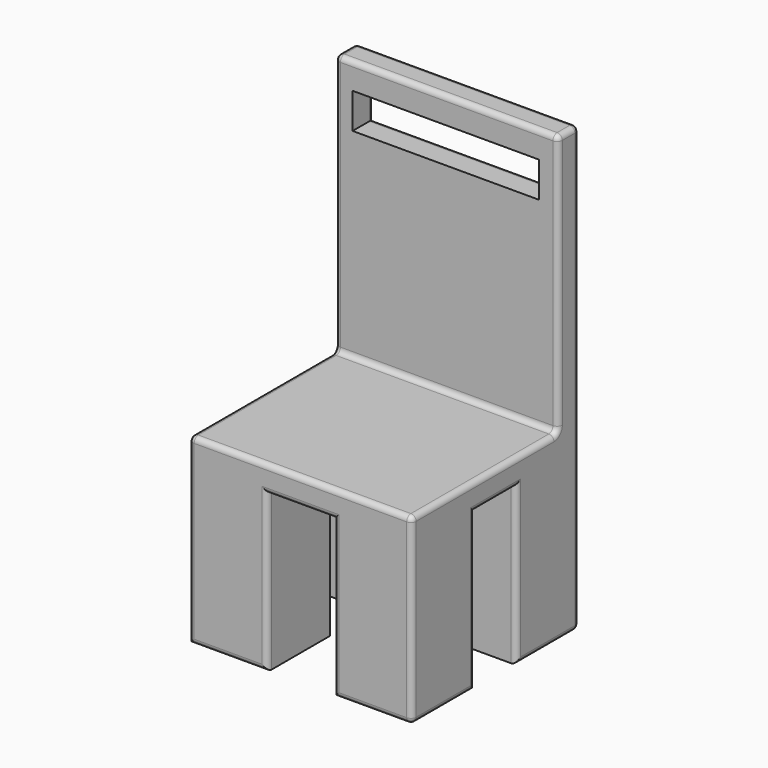
from build123d import *

# Parameters (mm, degrees)
F0_W     = 15
F0_H     = 15
F1_DEPTH = 30
F2_W     = 42.7
F2_H     = 40
F3_DEPTH = 5
F4_W     = 42.7
F4_H     = 5
F5_DEPTH = 50
F6_W     = 35.6923062354
F6_H     = 6.7692324519
F7_DEPTH = 25
F8_R     = 1


with BuildPart() as f1:
    # F0 (on Top) → F1 (new body)
    with BuildSketch(Plane.XY):
        with Locations((17.5, 17.5)):
            Rectangle(F0_W, F0_H)
    extrude(amount=F1_DEPTH)



with BuildPart() as f1b:
    # F0 (on Top) → F1, piece 2 (new body)
    with BuildSketch(Plane.XY):
        with Locations((17.5, 42.5)):
            Rectangle(F0_W, F0_H)
    extrude(amount=F1_DEPTH)


with BuildPart() as f1c:
    # F0 (on Top) → F1, piece 3 (new body)
    with BuildSketch(Plane.XY):
        with Locations((45.2, 17.5)):
            Rectangle(F0_W, F0_H)
    extrude(amount=F1_DEPTH)


with BuildPart() as f1d:
    # F0 (on Top) → F1, piece 4 (new body)
    with BuildSketch(Plane.XY):
        with Locations((45.2, 42.5)):
            Rectangle(F0_W, F0_H)
    extrude(amount=F1_DEPTH)


with BuildPart() as f1_1:
    add(f1.part)

    add(f1b.part)  # F3 merges F1b

    add(f1c.part)  # F3 merges F1c

    add(f1d.part)  # F3 merges F1d
    # F2 (on face) → F3 (join)
    with BuildSketch(Plane.XY.offset(30)):
        with Locations((31.35, 30)):
            Rectangle(F2_W, F2_H)
    extrude(amount=F3_DEPTH)

    # F4 (on face) → F5 (join)
    with BuildSketch(Plane.XY.offset(35)):
        with Locations((31.35, 47.5)):
            Rectangle(F4_W, F4_H)
    extrude(amount=F5_DEPTH)

    # F6 (on face) → F7 (cut)
    with BuildSketch(Plane(origin=(0, 50, 0), x_dir=(-1, 0, 0), z_dir=(0, 1, 0))):
        with Locations((-31.1794867739, 76.5897445381)):
            Rectangle(F6_W, F6_H)
    extrude(amount=-F7_DEPTH, mode=Mode.SUBTRACT)

    # F8
    f8_edges = [f1_1.edges().sort_by_distance(p)[0] for p in [
        (52.7, 27.5, 35),
        (31.35, 10, 35),
        (10, 27.5, 35),
        (31.35, 45, 35),
        (31.35, 50, 85),
        (10, 47.5, 85),
        (31.35, 45, 85),
        (52.7, 47.5, 85),
        (37.7, 10, 15),
        (31.35, 10, 30),
        (25, 10, 15),
        (17.5, 10, 0),
        (10, 10, 17.5),
        (52.7, 10, 17.5),
        (45.2, 10, 0),
        (52.7, 35, 15),
        (52.7, 30, 30),
        (52.7, 25, 15),
        (52.7, 17.5, 0),
        (52.7, 45, 60),
        (52.7, 50, 42.5),
        (52.7, 42.5, 0),
        (45.2, 50, 0),
        (10, 50, 42.5),
        (37.7, 50, 15),
        (17.5, 50, 0),
        (31.35, 50, 30),
        (25, 50, 15),
        (13.333334, 50, 76.589745),
        (31.179487, 50, 73.205128),
        (49.02564, 50, 76.589745),
        (31.179487, 50, 79.974361),
        (10, 45, 60),
    ]]
    fillet(f8_edges, radius=F8_R)


solid = f1_1.part
